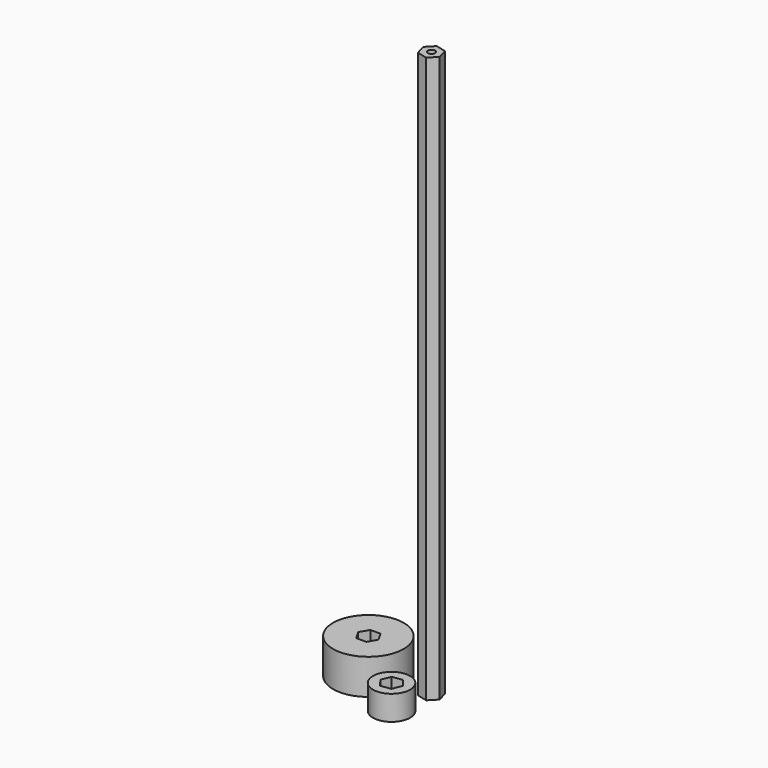
from build123d import *

# Parameters (mm, degrees)
F2_R     = 25.4
F3_DEPTH = 25.4
F4_R     = 2.5527
F5_DEPTH = 406.4
F6_R     = 13.3424155759
F7_DEPTH = 17.78


# Not quite as in the source:
# - a variable given as a bare number and used for a length is read in inches; the dataset says mm whatever the document's units were


with BuildPart() as f3:
    # F2 (on Top) → F3 (new body)
    with BuildSketch(Plane.XY):
        with Locations((-80.6699842215, 51.2332357466)):
            Circle(F2_R)
        Polygon((-73.3376358028, 51.2332357466), (-77.0038100121, 44.8832357466), (-84.3361584308, 44.8832357466), (-88.0023326402, 51.2332357466), (-84.3361584308, 57.5832357466), (-77.0038100121, 57.5832357466), align=None, mode=Mode.SUBTRACT)
    extrude(amount=F3_DEPTH)


with BuildPart() as f5:
    # F4 (on Top) → F5 (new body)
    with BuildSketch(Plane.XY):
        Polygon((-36.9019653495, 48.4404217775), (-31.6012177704, 53.9239544898), (-33.6997226121, 61.2563029085), (-41.098975033, 63.1051186149), (-46.3997226121, 57.6215859026), (-44.3012177704, 50.2892374839), align=None)
        with Locations((-39.0004701912, 55.7727701962)):
            Circle(F4_R, mode=Mode.SUBTRACT)
    extrude(amount=F5_DEPTH)


with BuildPart() as f7:
    # F6 (on Top) → F7 (new body)
    with BuildSketch(Plane.XY):
        with Locations((-44.0439581871, 26.2740552425)):
            Circle(F6_R)
        Polygon((-36.785788924, 27.3143976291), (-39.5139106202, 20.508467469), (-46.7720798833, 19.4681250824), (-51.3021274502, 25.233712856), (-48.5740057541, 32.0396430161), (-41.3158364909, 33.0799854026), align=None, mode=Mode.SUBTRACT)
    extrude(amount=F7_DEPTH)


solid = Compound([f3.part, f5.part, f7.part])
